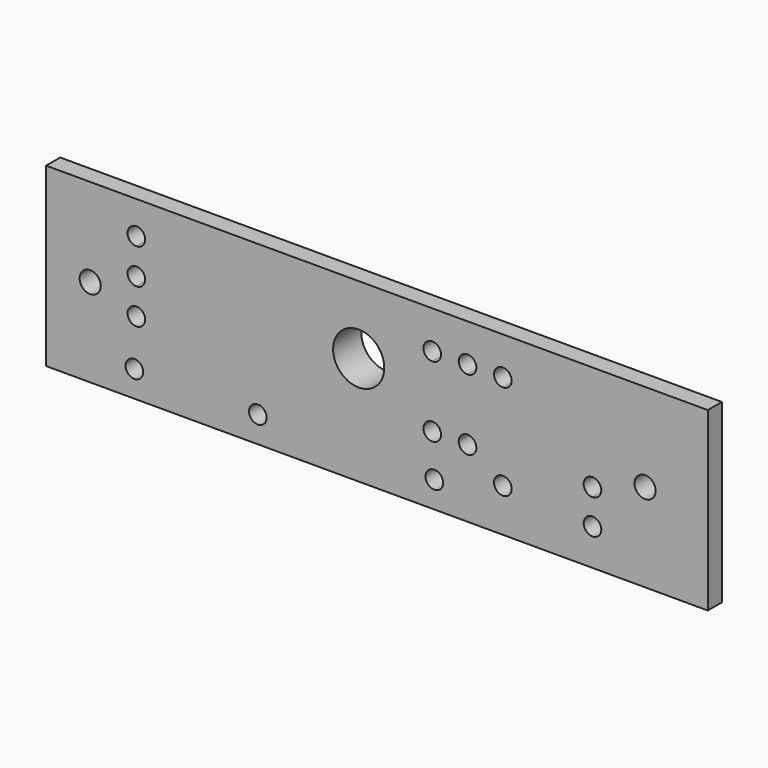
from build123d import *

# Parameters (mm, degrees)
F0_R        = 0.635
F0_R_2      = 0.762
F1_DEPTH    = 2.54
F2_T1_DEPTH = 19.2320747894
F2_T3_DEPTH = 54.1570747894


# Not quite as in the source:
# - a fillet or chamfer that OpenCascade refuses, or shapes differently, is made with other operations: its cross-section is extruded or revolved along the edge and cut away or added


with BuildPart() as f1:
    # F0 (on Front) → F1 (new body)
    with BuildSketch(Plane.XZ):
        Polygon((44.45, 12.7), (0, 12.7), (-3.175, 12.7), (-3.175, 0), (0, 0), (44.45, 0), align=None)
        with Locations((3.1763850711, 1.8884516321)):
            Circle(F0_R, mode=Mode.SUBTRACT)
        with BuildLine():
            ThreePointArc((12.7013850711, 1.8884516321), (12.0663850711, 1.2534516321), (11.4313850711, 1.8884516321))
            ThreePointArc((11.4313850711, 1.8884516321), (12.0663850711, 2.5234516321), (12.7013850711, 1.8884516321))
        make_face(mode=Mode.SUBTRACT)
        with Locations((0, 6.35)):
            Circle(F0_R_2, mode=Mode.SUBTRACT)
        with BuildLine():
            ThreePointArc((3.9569724428, 5.2575343288), (2.8729596367, 4.8085215228), (3.3219724428, 5.8925343288))
            ThreePointArc((3.3219724428, 5.8925343288), (3.7709852488, 5.7065471349), (3.9569724428, 5.2575343288))
        make_face(mode=Mode.SUBTRACT)
        with BuildLine():
            ThreePointArc((25.4013850711, 1.8884516321), (24.7663850711, 1.2534516321), (24.1313850711, 1.8884516321))
            ThreePointArc((24.1313850711, 1.8884516321), (24.7663850711, 2.5234516321), (25.4013850711, 1.8884516321))
        make_face(mode=Mode.SUBTRACT)
        with BuildLine():
            ThreePointArc((30.3330272979, 3.1118398262), (29.2490144918, 2.6628270202), (29.6980272979, 3.7468398262))
            ThreePointArc((29.6980272979, 3.7468398262), (30.1470401039, 3.5608526323), (30.3330272979, 3.1118398262))
        make_face(mode=Mode.SUBTRACT)
        with BuildLine():
            ThreePointArc((36.7843080854, 2.629004186), (35.7002952794, 2.17999138), (36.1493080854, 3.264004186))
            ThreePointArc((36.1493080854, 3.264004186), (36.5983208915, 3.0780169921), (36.7843080854, 2.629004186))
        make_face(mode=Mode.SUBTRACT)
        with BuildLine():
            ThreePointArc((25.2530272979, 4.8898398262), (24.1690144918, 4.4408270202), (24.6180272979, 5.5248398262))
            ThreePointArc((24.6180272979, 5.5248398262), (25.0670401039, 5.3388526323), (25.2530272979, 4.8898398262))
        make_face(mode=Mode.SUBTRACT)
        with BuildLine():
            ThreePointArc((27.7930272979, 4.8898398262), (27.1580272979, 4.2548398262), (26.5230272979, 4.8898398262))
            ThreePointArc((26.5230272979, 4.8898398262), (26.7090144918, 5.3388526323), (27.1580272979, 5.5248398262))
            ThreePointArc((27.1580272979, 5.5248398262), (27.6070401039, 5.3388526323), (27.7930272979, 4.8898398262))
        make_face(mode=Mode.SUBTRACT)
        with BuildLine():
            ThreePointArc((36.7843080854, 5.118204186), (36.5983208915, 4.66919138), (36.1493080854, 4.483204186))
            ThreePointArc((36.1493080854, 4.483204186), (35.7002952794, 5.5672169921), (36.7843080854, 5.118204186))
        make_face(mode=Mode.SUBTRACT)
        with Locations((39.9367623031, 6.35)):
            Circle(F0_R_2, mode=Mode.SUBTRACT)
        with BuildLine():
            ThreePointArc((3.3219724428, 7.1625343288), (2.6869724428, 7.7975343288), (3.3219724428, 8.4325343288))
            ThreePointArc((3.3219724428, 8.4325343288), (3.7709852488, 8.2465471349), (3.9569724428, 7.7975343288))
            ThreePointArc((3.9569724428, 7.7975343288), (3.7709852488, 7.3485215228), (3.3219724428, 7.1625343288))
        make_face(mode=Mode.SUBTRACT)
        with BuildLine():
            ThreePointArc((21.1654724428, 7.7975343288), (19.3239724428, 5.9560343288), (17.4824724428, 7.7975343288))
            ThreePointArc((17.4824724428, 7.7975343288), (19.3239724428, 9.6390343288), (21.1654724428, 7.7975343288))
        make_face(mode=Mode.SUBTRACT)
        with BuildLine():
            ThreePointArc((3.3219724428, 9.7025343288), (2.8729596367, 10.7865471349), (3.9569724428, 10.3375343288))
            ThreePointArc((3.9569724428, 10.3375343288), (3.7709852488, 9.8885215228), (3.3219724428, 9.7025343288))
        make_face(mode=Mode.SUBTRACT)
        with BuildLine():
            ThreePointArc((25.2530272979, 9.9698398262), (25.0670401039, 9.5208270202), (24.6180272979, 9.3348398262))
            ThreePointArc((24.6180272979, 9.3348398262), (24.1690144918, 10.4188526323), (25.2530272979, 9.9698398262))
        make_face(mode=Mode.SUBTRACT)
        with BuildLine():
            ThreePointArc((27.7930272979, 9.9698398262), (27.6070401039, 9.5208270202), (27.1580272979, 9.3348398262))
            ThreePointArc((27.1580272979, 9.3348398262), (26.7090144918, 10.4188526323), (27.7930272979, 9.9698398262))
        make_face(mode=Mode.SUBTRACT)
        with BuildLine():
            ThreePointArc((29.6980272979, 9.3348398262), (29.2490144918, 9.5208270202), (29.0630272979, 9.9698398262))
            ThreePointArc((29.0630272979, 9.9698398262), (29.6980272979, 10.6048398262), (30.3330272979, 9.9698398262))
            ThreePointArc((30.3330272979, 9.9698398262), (30.1470401039, 9.5208270202), (29.6980272979, 9.3348398262))
        make_face(mode=Mode.SUBTRACT)
    extrude(amount=F1_DEPTH)

    # F2: chamfer of 1.27 on 4 edges, made by hand

    # F2_s2 → F2_t1 (cut)
    with BuildSketch(Plane.XY.offset(-3.2660373947)):
        Polygon((43.18, 0), (44.45, -1.27), (44.45, 0), align=None)
        Polygon((-1.905, 0), (-3.175, -1.27), (-3.175, 0), align=None)
    extrude(amount=F2_T1_DEPTH, mode=Mode.SUBTRACT)

    # F2_s4 → F2_t3 (cut)
    with BuildSketch(Plane.YZ.offset(-6.4410373947)):
        Polygon((-1.27, 12.7), (0, 11.43), (0, 12.7), align=None)
        Polygon((0, 1.27), (-1.27, 0), (0, 0), align=None)
    extrude(amount=F2_T3_DEPTH, mode=Mode.SUBTRACT)


solid = f1.part
